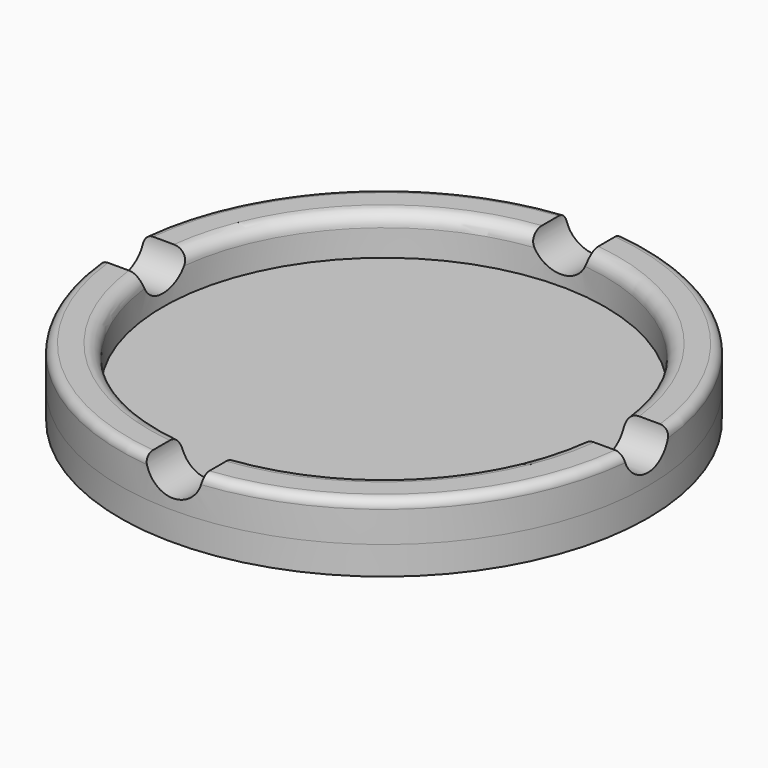
from build123d import *

# Parameters (mm, degrees)
F0_R         = 75.9313176518
F0_R_2       = 63.6217413668
F1_DEPTH     = 8.128
F2_DEPTH     = 11.43
F3_R         = 8.1097941577
F4_DEPTH     = 100.33
F5_DEPTH     = 117.094
F6_R         = 8.1153
F7_DEPTH     = 85.852
F8_DEPTH     = 117.094
F9_T2_ANGLE  = 87.3226513318
F9_T4_ANGLE  = 87.3226513318
F9_T6_ANGLE  = 87.3226513318
F9_T8_ANGLE  = 87.3226513318
F10_T2_ANGLE = 92.5127162525
F10_T4_ANGLE = 92.5127162525
F10_T6_ANGLE = 92.5127162525
F10_T8_ANGLE = 92.5127162525


# Not quite as in the source:
# - a fillet or chamfer that OpenCascade refuses, or shapes differently, is made with other operations: its cross-section is extruded or revolved along the edge and cut away or added


with BuildPart() as f1:
    # F0 (on Top) → F1 (new body)
    with BuildSketch(Plane.XY):
        Circle(F0_R)
        Circle(F0_R_2, mode=Mode.SUBTRACT)
        Circle(F0_R_2)
    extrude(amount=-F1_DEPTH)

    # F0 (on Top) → F2 (join)
    with BuildSketch(Plane.XY):
        Circle(F0_R)
        Circle(F0_R_2, mode=Mode.SUBTRACT)
    extrude(amount=F2_DEPTH)

    # F3 (on Right) → F4 (cut)
    with BuildSketch(Plane.YZ):
        with Locations((0, 11.5122310817)):
            Circle(F3_R)
    extrude(amount=-F4_DEPTH, mode=Mode.SUBTRACT)

    # F3 (on Right) → F5 (cut)
    with BuildSketch(Plane.YZ):
        with Locations((0, 11.5122310817)):
            Circle(F3_R)
    extrude(amount=F5_DEPTH, mode=Mode.SUBTRACT)

    # F6 (on Front) → F7 (cut)
    with BuildSketch(Plane.XZ):
        with Locations((0, 11.1844760826)):
            Circle(F6_R)
    extrude(amount=-F7_DEPTH, mode=Mode.SUBTRACT)

    # F6 (on Front) → F8 (cut, symmetric)
    with BuildSketch(Plane.XZ):
        with Locations((0, 11.1844760826)):
            Circle(F6_R)
    extrude(amount=F8_DEPTH, both=True, mode=Mode.SUBTRACT)

    # F9: fillet of radius 2.54 on 4 edges, made by hand

    # F9_s1 → F9_t2 (revolve, cut)
    with BuildSketch(Plane(origin=(0, 0, 0), x_dir=(0, 0, 1), z_dir=(-0.999726726, -0.0233767669, 0))):
        with BuildLine():
            ThreePointArc((8.89, -75.9313176518), (10.6860512242, -75.187368876), (11.43, -73.3913176518))
            Line((11.43, -73.3913176518), (11.43, -75.9313176518))
            Line((11.43, -75.9313176518), (8.89, -75.9313176518))
        make_face()
    revolve(axis=Axis((0, 0, 11.43), (0, 0, 1)), revolution_arc=F9_T2_ANGLE, mode=Mode.SUBTRACT)

    # F9_s3 → F9_t4 (revolve, cut)
    with BuildSketch(Plane(origin=(0, 0, 0), x_dir=(0, 0, 1), z_dir=(-0.0233475312, 0.9997274092, 0))):
        with BuildLine():
            ThreePointArc((8.89, -75.9313176518), (10.6860512242, -75.187368876), (11.43, -73.3913176518))
            Line((11.43, -73.3913176518), (11.43, -75.9313176518))
            Line((11.43, -75.9313176518), (8.89, -75.9313176518))
        make_face()
    revolve(axis=Axis((0, 0, 11.43), (0, 0, 1)), revolution_arc=F9_T4_ANGLE, mode=Mode.SUBTRACT)

    # F9_s5 → F9_t6 (revolve, cut)
    with BuildSketch(Plane(origin=(0, 0, 0), x_dir=(0, 0, 1), z_dir=(0.999726726, 0.0233767669, 0))):
        with BuildLine():
            ThreePointArc((8.89, -75.9313176518), (10.6860512242, -75.187368876), (11.43, -73.3913176518))
            Line((11.43, -73.3913176518), (11.43, -75.9313176518))
            Line((11.43, -75.9313176518), (8.89, -75.9313176518))
        make_face()
    revolve(axis=Axis((0, 0, 11.43), (0, 0, 1)), revolution_arc=F9_T6_ANGLE, mode=Mode.SUBTRACT)

    # F9_s7 → F9_t8 (revolve, cut)
    with BuildSketch(Plane(origin=(0, 0, 0), x_dir=(0, 0, 1), z_dir=(0.0233475312, -0.9997274092, 0))):
        with BuildLine():
            ThreePointArc((8.89, -75.9313176518), (10.6860512242, -75.187368876), (11.43, -73.3913176518))
            Line((11.43, -73.3913176518), (11.43, -75.9313176518))
            Line((11.43, -75.9313176518), (8.89, -75.9313176518))
        make_face()
    revolve(axis=Axis((0, 0, 11.43), (0, 0, 1)), revolution_arc=F9_T8_ANGLE, mode=Mode.SUBTRACT)

    # F10: fillet of radius 3.81 on 4 edges, made by hand

    # F10_s1 → F10_t2 (revolve, cut)
    with BuildSketch(Plane(origin=(0, 0, 0), x_dir=(0, 0, 1), z_dir=(-0.9997599835, 0.0219083392, 0))):
        with BuildLine():
            ThreePointArc((11.43, -67.4317413668), (10.3140768363, -64.7376645305), (7.62, -63.6217413668))
            Line((7.62, -63.6217413668), (11.43, -63.6217413668))
            Line((11.43, -63.6217413668), (11.43, -67.4317413668))
        make_face()
    revolve(axis=Axis((0, 0, 11.43), (0, 0, 1)), revolution_arc=F10_T2_ANGLE, mode=Mode.SUBTRACT)

    # F10_s3 → F10_t4 (revolve, cut)
    with BuildSketch(Plane(origin=(0, 0, 0), x_dir=(0, 0, 1), z_dir=(-0.0219433183, -0.9997592164, 0))):
        with BuildLine():
            ThreePointArc((7.62, -63.6217413668), (10.3140768363, -64.7376645305), (11.43, -67.4317413668))
            Line((11.43, -67.4317413668), (11.43, -63.6217413668))
            Line((11.43, -63.6217413668), (7.62, -63.6217413668))
        make_face()
    revolve(axis=Axis((0, 0, 11.43), (0, 0, 1)), revolution_arc=F10_T4_ANGLE, mode=Mode.SUBTRACT)

    # F10_s5 → F10_t6 (revolve, cut)
    with BuildSketch(Plane(origin=(0, 0, 0), x_dir=(0, 0, 1), z_dir=(0.9997599835, -0.0219083392, 0))):
        with BuildLine():
            ThreePointArc((7.62, -63.6217413668), (10.3140768363, -64.7376645305), (11.43, -67.4317413668))
            Line((11.43, -67.4317413668), (11.43, -63.6217413668))
            Line((11.43, -63.6217413668), (7.62, -63.6217413668))
        make_face()
    revolve(axis=Axis((0, 0, 11.43), (0, 0, 1)), revolution_arc=F10_T6_ANGLE, mode=Mode.SUBTRACT)

    # F10_s7 → F10_t8 (revolve, cut)
    with BuildSketch(Plane(origin=(0, 0, 0), x_dir=(0, 0, 1), z_dir=(0.0219433183, 0.9997592164, 0))):
        with BuildLine():
            ThreePointArc((7.62, -63.6217413668), (10.3140768363, -64.7376645305), (11.43, -67.4317413668))
            Line((11.43, -67.4317413668), (11.43, -63.6217413668))
            Line((11.43, -63.6217413668), (7.62, -63.6217413668))
        make_face()
    revolve(axis=Axis((0, 0, 11.43), (0, 0, 1)), revolution_arc=F10_T8_ANGLE, mode=Mode.SUBTRACT)


solid = f1.part
